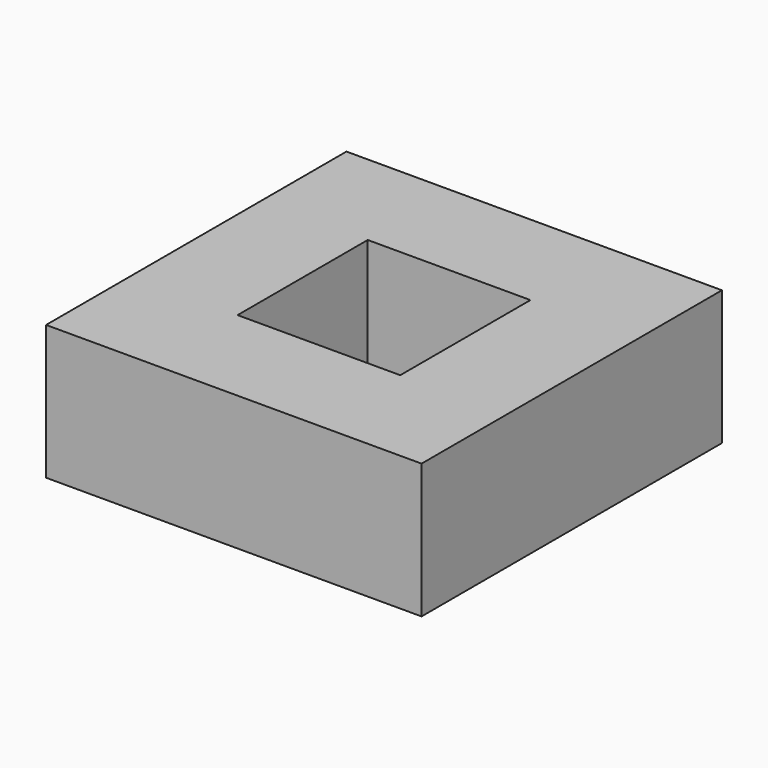
from build123d import *

# Parameters (mm, degrees)
F0_W     = 120
F0_H     = 120
F1_DEPTH = 3
F2_W     = 52
F2_H     = 52
F3_DEPTH = 25
F2_W_2   = 120
F2_H_2   = 120
F2_W_3   = 70
F2_H_3   = 70
F2_R     = 2.5
F4_DEPTH = 37
F5_W     = 120
F5_H     = 120
F5_W_2   = 114
F5_H_2   = 114
F5_W_3   = 52
F5_H_3   = 52
F6_DEPTH = 3


with BuildPart() as f1:
    # F0 (on Top) → F1 (new body)
    with BuildSketch(Plane.XY):
        Rectangle(F0_W, F0_H)
    extrude(amount=F1_DEPTH)

    # F2 (on face) → F3 (cut)
    with BuildSketch(Plane.XY.offset(3)):
        Rectangle(F2_W, F2_H)
    extrude(amount=-F3_DEPTH, mode=Mode.SUBTRACT)

    # F2 (on face) → F4 (join)
    with BuildSketch(Plane.XY.offset(3)):
        Rectangle(F2_W_2, F2_H_2)
        Polygon((-57, -57), (-57, -35), (-57, 35), (-57, 57), (-35, 57), (35, 57), (57, 57), (57, 35), (57, -35), (57, -57), (35, -57), (-35, -57), align=None, mode=Mode.SUBTRACT)
        Rectangle(F2_W_3, F2_H_3)
        Rectangle(F2_W, F2_H, mode=Mode.SUBTRACT)
        with Locations((46, 46)):
            Circle(F2_R)
        with Locations((0, 46)):
            Circle(F2_R)
        with Locations((-46, 46)):
            Circle(F2_R)
        with Locations((-46, 0)):
            Circle(F2_R)
        with Locations((-46, -46)):
            Circle(F2_R)
        with Locations((0, -46)):
            Circle(F2_R)
        with Locations((46, -46)):
            Circle(F2_R)
        with Locations((46, 0)):
            Circle(F2_R)
    extrude(amount=F4_DEPTH)

    # F5 (on face) → F6 (join)
    with BuildSketch(Plane.XY.offset(40)):
        Rectangle(F5_W, F5_H)
        Rectangle(F5_W_2, F5_H_2, mode=Mode.SUBTRACT)
        Rectangle(F5_W_2, F5_H_2)
        Rectangle(F5_W_3, F5_H_3, mode=Mode.SUBTRACT)
    extrude(amount=F6_DEPTH)


solid = f1.part
